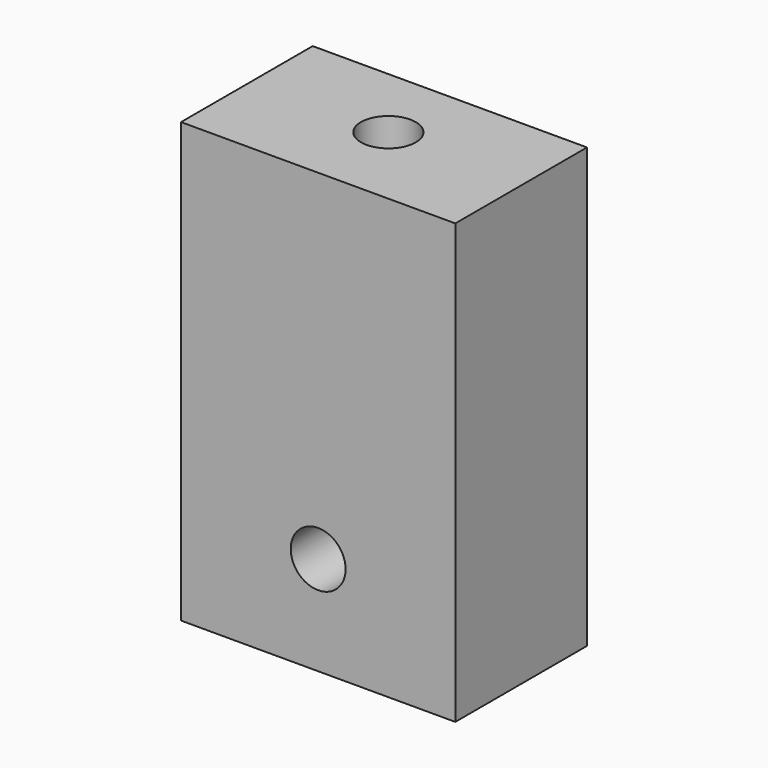
from build123d import *
from build123d import SkipClean  # not in build123d's __all__

# Parameters (mm, degrees)
F0_W     = 50
F0_H     = 80
F1_DEPTH = 30
F2_R     = 5
F3_DEPTH = 20
F4_R     = 5
F5_DEPTH = 25
F6_R     = 5
F7_DEPTH = 65


with BuildPart() as f1:
    # F0 (on Front) → F1 (new body)
    with BuildSketch(Plane.XZ):
        with Locations((0, 40)):
            Rectangle(F0_W, F0_H)
    extrude(amount=F1_DEPTH)

    # F2 (on face) → F3 (cut)
    with BuildSketch(Plane.XZ.offset(30)):
        with Locations((0, 18)):
            Circle(F2_R)
    extrude(amount=-F3_DEPTH, mode=Mode.SUBTRACT)

    # F4 (on face) → F5 (cut)
    with BuildSketch(Plane(origin=(-25, 0, 0), x_dir=(0, -1, 0), z_dir=(-1, 0, 0))):
        with Locations((16, 18)):
            Circle(F4_R)
    extrude(amount=-F5_DEPTH, mode=Mode.SUBTRACT)

    # F6 (on face) → F7 (cut)
    with BuildSketch(Plane.XY.offset(80)):
        with Locations((0, -14)):
            Circle(F6_R)
    with SkipClean():  # cleaning this boolean's faces spoils the solid; the shape is the same uncleaned
        extrude(amount=-F7_DEPTH, mode=Mode.SUBTRACT)


solid = f1.part
